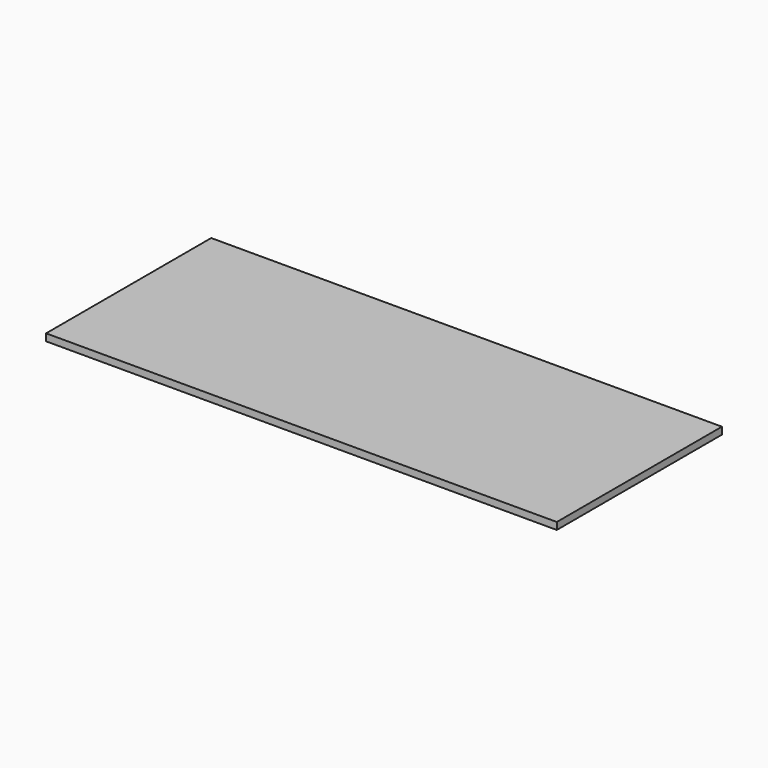
from build123d import *

# Parameters (mm, degrees)
F0_TEXT_SIZE = 28.0260186022
F1_DEPTH     = 3.175
F2_W         = 230.0757961348
F2_H         = 92.9840020835
F3_DEPTH     = 3.175


# Not quite as in the source:
# - Text() gives the source's letters only with a copy of the font that has no kerning and outlines rounded to 1/6400 em; it was checked with that copy


with BuildPart() as f1:
    # F0 (on Top) → F1 (new body)
    with BuildSketch(Plane.XY):
        with Locations((0, 0)):
            Text('Stuck with me', F0_TEXT_SIZE, font='Open Sans', font_style=FontStyle.BOLD, text_align=(TextAlign.LEFT, TextAlign.BOTTOM))
        with Locations((0, -38.1153852989)):
            Text('now, shithead', F0_TEXT_SIZE, font='Open Sans', font_style=FontStyle.BOLD, text_align=(TextAlign.LEFT, TextAlign.BOTTOM))
    extrude(amount=F1_DEPTH)


with BuildPart() as f3:
    # F2 (on face) → F3 (new body)
    with BuildSketch(Plane.XY.offset(3.175)):
        with Locations((100.4170677625, -12.3196598142)):
            Rectangle(F2_W, F2_H)
    extrude(amount=F3_DEPTH)


solid = Compound([f1.part, f3.part])
